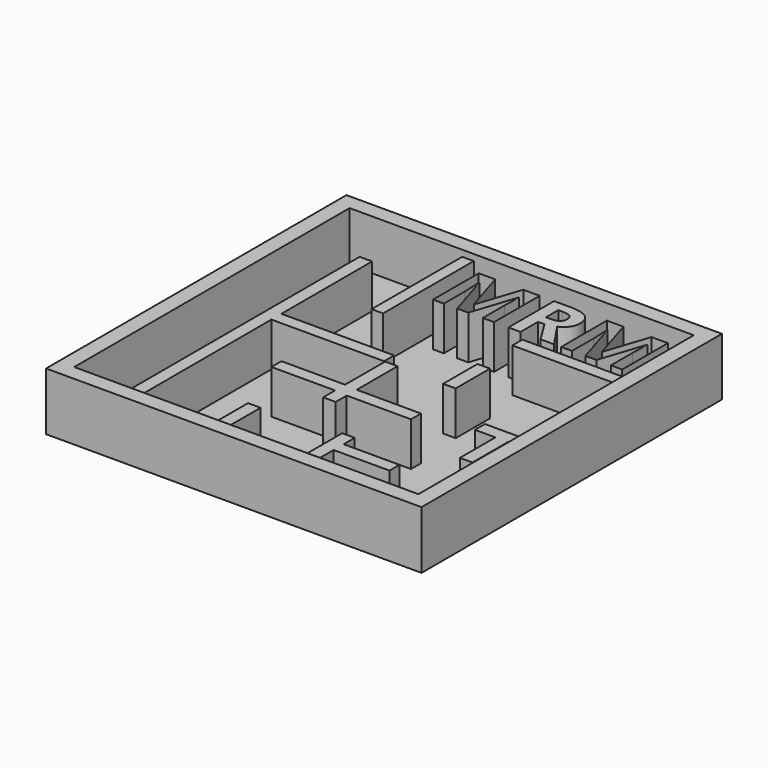
from build123d import *

# Parameters (mm, degrees)
F0_W         = 38.1
F0_H         = 38.1
F1_DEPTH     = 0.79375
F2_W         = 38.1
F2_H         = 38.1
F2_W_2       = 34.925
F2_H_2       = 34.925
F3_DEPTH     = 5.08
F4_W         = 1.27
F4_H         = 4.7155919945
F4_H_2       = 4.3553267606
F5_DEPTH     = 4.445
F4_TEXT_SIZE = 8.1138888889
F6_DEPTH     = 4.445
F7_R         = 1.27
F8_DEPTH     = 0.396875


# Not quite as in the source:
# - a feature names something its author has since deleted; it is built from what else it names
# - Text() gives the source's letters only with a copy of the font that has no kerning and outlines rounded to 1/6400 em; it was checked with that copy


with BuildPart() as f1:
    # F0 (on Top) → F1 (new body)
    with BuildSketch(Plane.XY):
        with Locations((-0.9589064866, 4.2466382542)):
            Rectangle(F0_W, F0_H)
    extrude(amount=-F1_DEPTH)

    # F2 (on face) → F3 (join)
    with BuildSketch(Plane.XY):
        with Locations((-0.9589064866, 4.2466382542)):
            Rectangle(F2_W, F2_H)
        with Locations((-0.9589064866, 4.2466382542)):
            Rectangle(F2_W_2, F2_H_2, mode=Mode.SUBTRACT)
    extrude(amount=F3_DEPTH)

    # F4 (on face) → F5 (join)
    with BuildSketch(Plane.XY):
        Polygon((-5.8208061878, 21.7091382542), (-6.9914064866, 21.7091382542), (-6.9914064866, 10.205207935), (-5.8208061878, 10.205207935), (-5.8208061878, 15.8923946853), (-5.8208061878, 16.2254381761), align=None)
        Polygon((15.6901365114, -0.8429788161), (16.5035935134, -0.8429788161), (16.5035935134, 0.4270211839), (12.3366795094, 0.4270211839), (12.3366795094, -0.8429788161), (14.4201365114, -0.8429788161), (14.4201365114, -5.3423652425), (15.6901365114, -5.3423652425), align=None)
        Polygon((4.4872411527, -7.8667792624), (4.4872411527, -13.2158617458), (5.7572411527, -13.2158617458), (5.7572411527, -10.5413205041), (11.4235935134, -10.5413205041), (11.4235935134, -9.2713205041), (5.7572411527, -9.2713205041), (5.7572411527, -7.8667792624), align=None)
        with Locations((-3.9238879068, -10.8580657485)):
            Rectangle(F4_W, F4_H)
        with Locations((6.0773501715, 5.9274036559)):
            Rectangle(F4_W, F4_H_2)
        Polygon((16.5035935134, 12.3170964573), (16.5035935134, 13.5870964573), (9.4863983137, 13.5870964573), (8.2193944869, 13.5870964573), (5.6091938122, 13.5870964573), (5.6091938122, 12.3170964573), align=None)
        Polygon((-12.0714064866, 5.125207935), (-12.0714064866, 3.855207935), (-0.6367194497, 3.855207935), (-0.6367194497, 5.125207935), (-2.0346737001, 5.125207935), align=None)
        Polygon((-13.3414064866, 16.6291382542), (-13.3414064866, -13.2158617458), (-12.0714064866, -13.2158617458), (-12.0714064866, 3.855207935), (-12.0714064866, 5.125207935), (-12.0714064866, 16.6291382542), align=None)
    extrude(amount=F5_DEPTH)

    # F4 (on face) → F6 (join)
    with BuildSketch(Plane.XY):
        Polygon((-13.3414064866, 16.6291382542), (-13.3414064866, -13.2158617458), (-12.0714064866, -13.2158617458), (-12.0714064866, 3.855207935), (-12.0714064866, 5.125207935), (-12.0714064866, 16.6291382542), align=None)
        Polygon((0.7347630268, 3.855207935), (-0.5308500946, 3.855207935), (-0.5308500946, -1.224792065), (-6.9914064866, -1.224792065), (-6.9914064866, -2.494792065), (-0.5308500946, -2.494792065), (-0.5308500946, -4.0023759939), (0.7347630268, -4.0023759939), (0.7347630268, -2.6002597244), (7.2566795094, -2.6002597244), (7.2566795094, -1.3302597244), (5.8147630268, -1.3302597244), (5.7516207849, -1.3302597244), (0.7347630268, -1.3302597244), align=None)
        Polygon((-12.0714064866, 5.125207935), (-12.0714064866, 3.855207935), (-0.6367194497, 3.855207935), (-0.6367194497, 5.125207935), (-2.0346737001, 5.125207935), align=None)
        Polygon((-5.8208061878, 16.2254381761), (-5.8208061878, 21.7091382542), (-6.9914064866, 21.7091382542), (-6.9914064866, 10.205207935), (-5.8208061878, 10.205207935), (-5.8208061878, 15.8923946853), align=None)
        Polygon((15.6901365114, -0.8429788161), (16.5035935134, -0.8429788161), (16.5035935134, 0.4270211839), (12.3366795094, 0.4270211839), (12.3366795094, -0.8429788161), (14.4201365114, -0.8429788161), (14.4201365114, -5.3423652425), (15.6901365114, -5.3423652425), align=None)
        Polygon((4.4872411527, -7.8667792624), (4.4872411527, -13.2158617458), (5.7572411527, -13.2158617458), (5.7572411527, -10.5413205041), (11.4235935134, -10.5413205041), (11.4235935134, -9.2713205041), (5.7572411527, -9.2713205041), (5.7572411527, -7.8667792624), align=None)
        with Locations((-3.9238879068, -10.8580657485)):
            Rectangle(F4_W, F4_H)
        with Locations((6.0773501715, 5.9274036559)):
            Rectangle(F4_W, F4_H_2)
        Polygon((5.6091938122, 12.3170964573), (16.5035935134, 12.3170964573), (16.5035935134, 13.5870964573), (9.4863983137, 13.5870964573), (8.2193944869, 13.5870964573), (5.6091938122, 13.5870964573), align=None)
        with Locations((-4.9391339999, 14.5303609447)):
            Text('MRM', F4_TEXT_SIZE, font='Open Sans', font_style=FontStyle.BOLD, text_align=(TextAlign.LEFT, TextAlign.BOTTOM))
    extrude(amount=F6_DEPTH)

    # F7 (on face) → F8 (cut)
    with BuildSketch(Plane.XY):
        with Locations((-3.0708500946, 1.315207935)):
            Circle(F7_R)
        with Locations((-15.8814064866, -10.6758617458)):
            Circle(F7_R)
    extrude(amount=-F8_DEPTH, mode=Mode.SUBTRACT)


solid = f1.part
